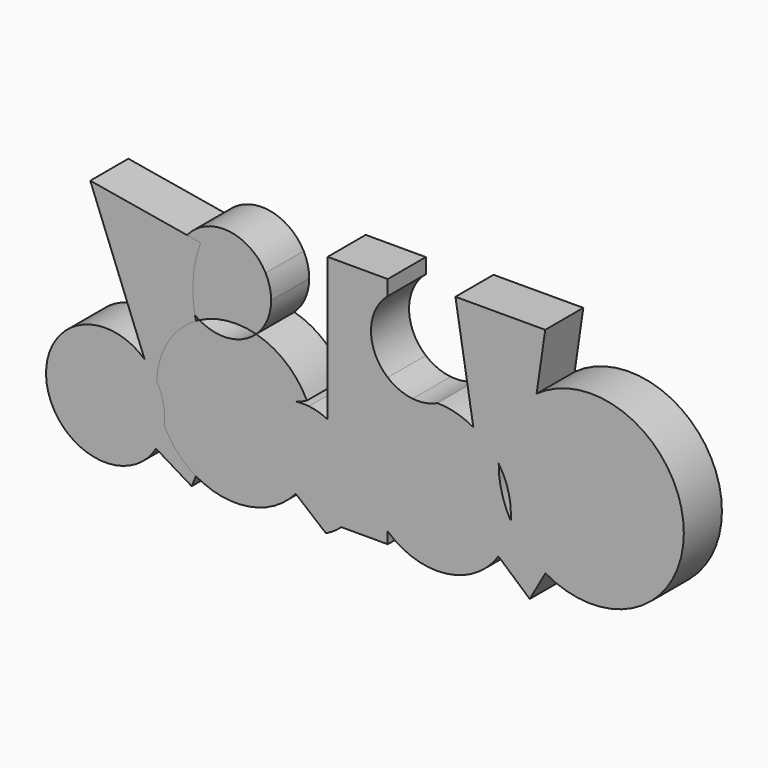
from build123d import *

# Parameters (mm, degrees)
F3_DEPTH = 25


with BuildPart() as f3:
    # F0 (on Front) → F3 (new body)
    with BuildSketch(Plane.XZ):
        with BuildLine():
            ThreePointArc((-57.5129599565, -16.0864628453), (-54.1744360224, -8.3492191036), (-53.0337243425, 0))
            ThreePointArc((-53.0337243425, 0), (-55.7869818002, 12.7989524029), (-63.5596679574, 23.3336075535))
            ThreePointArc((-63.5596679574, 23.3336075535), (-114.9250954512, -4.7192103171), (-57.5129599565, -16.0864628453))
        make_face()
        with BuildLine():
            ThreePointArc((-63.5596679574, 23.3336075535), (-55.7869818002, 12.7989524029), (-53.0337243425, 0))
            ThreePointArc((-53.0337243425, 0), (-54.1744360224, -8.3492191036), (-57.5129599565, -16.0864628453))
            Line((-57.5129599565, -16.0864628453), (-38.822568953, -27.3698866367))
            Line((-38.822568953, -27.3698866367), (-19.6386948228, 19.145950675))
            ThreePointArc((-19.6386948228, 19.145950675), (-30.9162562326, 34.4599627539), (-37.1640258454, 52.4229171927))
            ThreePointArc((-37.1640258454, 52.4229171927), (-46.7150991932, 69.3136234913), (-41.2417085605, 87.9297712223))
            Line((-41.2417085605, 87.9297712223), (-92.067733407, 96.5796262026))
            Line((-92.067733407, 96.5796262026), (-63.5596679574, 23.3336075535))
        make_face()
        with BuildLine():
            Line((-34.0956747532, 86.7136195302), (-41.2417085605, 87.9297712223))
            ThreePointArc((-41.2417085605, 87.9297712223), (-46.7150991932, 69.3136234913), (-37.1640258454, 52.4229171927))
            ThreePointArc((-37.1640258454, 52.4229171927), (-37.9931792296, 69.7797403469), (-34.0956747532, 86.7136195302))
        make_face()
    extrude(amount=F3_DEPTH)


with BuildPart() as f3b:
    # F1 (on face) → F3, piece 2 (new body)
    with BuildSketch(Plane.XZ):
        with BuildLine():
            ThreePointArc((22.6798846139, 29.6390745967), (19.3937151758, 29.8020017295), (16.1100178957, 29.5951515436))
            ThreePointArc((16.1100178957, 29.5951515436), (18.9410054417, 30.6292208692), (21.67584417, 31.895888539))
            ThreePointArc((21.67584417, 31.895888539), (10.7700522114, 45.849059237), (-4.9604636005, 53.9840542009))
            ThreePointArc((-4.9604636005, 53.9840542009), (-19.3186695983, 47.400145928), (-34.7485039853, 50.7804030796))
            ThreePointArc((-34.7485039853, 50.7804030796), (-35.6844274432, 50.2820713922), (-36.6073121526, 49.7599880627))
            ThreePointArc((-36.6073121526, 49.7599880627), (-30.2695427886, 33.2631947723), (-19.6386948228, 19.145950675))
            Line((-19.6386948228, 19.145950675), (-36.5888869277, -21.9537965919))
            ThreePointArc((-36.5888869277, -21.9537965919), (-8.7780666366, -27.0012589518), (15.8131210591, -13.0659767785))
            ThreePointArc((15.8131210591, -13.0659767785), (23.2066061979, -0.4695140568), (25.7772746795, 13.9084607363))
            ThreePointArc((25.7772746795, 13.9084607363), (24.9955637813, 21.9247884124), (22.6798846139, 29.6390745967))
        make_face()
        with BuildLine():
            ThreePointArc((32.5686484575, 26.7681818786), (27.7514826988, 28.6418231537), (22.6798846139, 29.6390745967))
            ThreePointArc((22.6798846139, 29.6390745967), (24.9955637813, 21.9247884124), (25.7772746795, 13.9084607363))
            ThreePointArc((25.7772746795, 13.9084607363), (23.2066061979, -0.4695140568), (15.8131210591, -13.0659767785))
            Line((15.8131210591, -13.0659767785), (31.6467881203, -26.148930192))
            ThreePointArc((31.6467881203, -26.148930192), (35.919117176, -23.7697035307), (39.7357987823, -20.712506026))
            Line((39.7357987823, -20.712506026), (32.5686484575, -20.712506026))
            Line((32.5686484575, -20.712506026), (32.5686484575, 26.7681818786))
        make_face()
        with BuildLine():
            Line((32.5686484575, 87.4569258152), (32.5686484575, 40.5099101671))
            ThreePointArc((32.5686484575, 40.5099101671), (41.2449777291, 63.9834179912), (32.5686484575, 87.4569258152))
        make_face()
        with BuildLine():
            ThreePointArc((32.5686484575, 87.4569258152), (41.2449777291, 63.9834179912), (32.5686484575, 40.5099101671))
            Line((32.5686484575, 40.5099101671), (32.5686484575, 26.7681818786))
            ThreePointArc((32.5686484575, 26.7681818786), (48.5364514198, 4.8972215897), (39.7357987823, -20.712506026))
            Line((39.7357987823, -20.712506026), (64.1396269202, -20.712506026))
            Line((64.1396269202, -20.712506026), (64.1396269202, -14.7266603521))
            ThreePointArc((64.1396269202, -14.7266603521), (51.1973866521, 14.2060667276), (64.1396269202, 43.1387938073))
            Line((64.1396269202, 43.1387938073), (64.1396269202, 56.3723585854))
            ThreePointArc((64.1396269202, 56.3723585854), (55.3361792801, 75.172799182), (64.1396269202, 93.9732397787))
            Line((64.1396269202, 93.9732397787), (64.1396269202, 101.8965914845))
            Line((64.1396269202, 101.8965914845), (32.5686484575, 101.8965914845))
            Line((32.5686484575, 101.8965914845), (32.5686484575, 87.4569258152))
        make_face()
        with BuildLine():
            ThreePointArc((39.7357987823, -20.712506026), (48.5364514198, 4.8972215897), (32.5686484575, 26.7681818786))
            Line((32.5686484575, 26.7681818786), (32.5686484575, -20.712506026))
            Line((32.5686484575, -20.712506026), (39.7357987823, -20.712506026))
        make_face()
        with BuildLine():
            ThreePointArc((-19.6386948228, 19.145950675), (-30.2695427886, 33.2631947723), (-36.6073121526, 49.7599880627))
            ThreePointArc((-36.6073121526, 49.7599880627), (-51.2845084466, 35.2785480536), (-57.1793476261, 15.5204341043))
            ThreePointArc((-57.1793476261, 15.5204341043), (-54.0879846732, 8.0322796764), (-53.0337243425, 0))
            ThreePointArc((-53.0337243425, 0), (-53.0907279184, -1.8828946308), (-53.261529853, -3.7588925779))
            ThreePointArc((-53.261529853, -3.7588925779), (-46.3091923785, -14.1245387359), (-36.5888869277, -21.9537965919))
            Line((-36.5888869277, -21.9537965919), (-19.6386948228, 19.145950675))
        make_face()
        with BuildLine():
            ThreePointArc((64.1396269202, 43.1387938073), (51.1973866521, 14.2060667276), (64.1396269202, -14.7266603521))
            Line((64.1396269202, -14.7266603521), (64.1396269202, 43.1387938073))
        make_face()
        with BuildLine():
            Line((64.1396269202, 43.1387938073), (64.1396269202, -14.7266603521))
            ThreePointArc((64.1396269202, -14.7266603521), (94.8714157265, -24.299133232), (122.2583204617, -7.3866369852))
            ThreePointArc((122.2583204617, -7.3866369852), (126.6693657888, 1.4672962095), (128.6989113378, 11.1487423185))
            ThreePointArc((128.6989113378, 11.1487423185), (123.9392055501, 22.9482151463), (122.4046294826, 35.578632182))
            ThreePointArc((122.4046294826, 35.578632182), (116.4841739619, 42.5844918046), (109.084925085, 48.0052831383))
            ThreePointArc((109.084925085, 48.0052831383), (99.9702550376, 51.7168828456), (90.2150532091, 53.0165827137))
            ThreePointArc((90.2150532091, 53.0165827137), (83.8500329286, 51.0314326127), (77.1854449114, 50.8376010994))
            ThreePointArc((77.1854449114, 50.8376010994), (70.2832808433, 47.6308544859), (64.1396269202, 43.1387938073))
        make_face()
        with BuildLine():
            Line((64.1396269202, 56.3723585854), (64.1396269202, 43.1387938073))
            ThreePointArc((64.1396269202, 43.1387938073), (70.2832808433, 47.6308544859), (77.1854449114, 50.8376010994))
            ThreePointArc((77.1854449114, 50.8376010994), (70.2532121523, 52.6401745495), (64.1396269202, 56.3723585854))
        make_face()
        with BuildLine():
            ThreePointArc((128.6989113378, 11.1487423185), (126.6693657888, 1.4672962095), (122.2583204617, -7.3866369852))
            Line((122.2583204617, -7.3866369852), (138.6857926846, -21.7697098851))
            Line((138.6857926846, -21.7697098851), (146.9266724857, -7.1460989624))
            ThreePointArc((146.9266724857, -7.1460989624), (136.5755240921, 0.7685904427), (128.6989113378, 11.1487423185))
        make_face()
        with BuildLine():
            Line((99.6706486582, 105.2629665375), (103.96512909, 79.1439118403))
            Line((103.96512909, 79.1439118403), (109.084925085, 48.0052831383))
            ThreePointArc((109.084925085, 48.0052831383), (116.4841739619, 42.5844918046), (122.4046294826, 35.578632182))
            ThreePointArc((122.4046294826, 35.578632182), (127.775402975, 57.2901740208), (142.2999815172, 74.2981978653))
            Line((142.2999815172, 74.2981978653), (146.8326449394, 105.3287759423))
            Line((146.8326449394, 105.3287759423), (99.6706486582, 105.2629665375))
        make_face()
        with BuildLine():
            ThreePointArc((128.8195184172, 14.2060667276), (128.789354926, 12.6762155412), (128.6989113378, 11.1487423185))
            ThreePointArc((128.6989113378, 11.1487423185), (136.5755240921, 0.7685904427), (146.9266724857, -7.1460989624))
            ThreePointArc((146.9266724857, -7.1460989624), (195.4224488753, -6.9551665697), (219.6153865573, 35.0755192339))
            ThreePointArc((219.6153865573, 35.0755192339), (192.9993129943, 78.4232134504), (142.2999815172, 74.2981978653))
            ThreePointArc((142.2999815172, 74.2981978653), (127.775402975, 57.2901740208), (122.4046294826, 35.578632182))
            ThreePointArc((122.4046294826, 35.578632182), (127.1812180547, 25.3633217008), (128.8195184172, 14.2060667276))
        make_face()
    extrude(amount=F3_DEPTH)


with BuildPart() as f3c:
    # F1 (on face) → F3, piece 3 (new body)
    with BuildSketch(Plane.XZ):
        with BuildLine():
            ThreePointArc((-34.7485039853, 50.7804030796), (-20.1537146111, 55.1645227662), (-4.9604636005, 53.9840542009))
            ThreePointArc((-4.9604636005, 53.9840542009), (0.8620484172, 62.252275739), (2.9158330555, 72.1541494131))
            ThreePointArc((2.9158330555, 72.1541494131), (2.1758787307, 78.1788806293), (0, 83.8454907605))
            ThreePointArc((0, 83.8454907605), (-19.5273271661, 96.9297048561), (-41.2417085605, 87.9297712223))
            Line((-41.2417085605, 87.9297712223), (-34.0956747532, 86.7136195302))
            ThreePointArc((-34.0956747532, 86.7136195302), (-37.9931792296, 69.7797403469), (-37.1640258454, 52.4229171927))
            ThreePointArc((-37.1640258454, 52.4229171927), (-35.9803745824, 51.5662038637), (-34.7485039853, 50.7804030796))
        make_face()
    extrude(amount=F3_DEPTH)


solid = Compound([f3.part, f3b.part, f3c.part])
